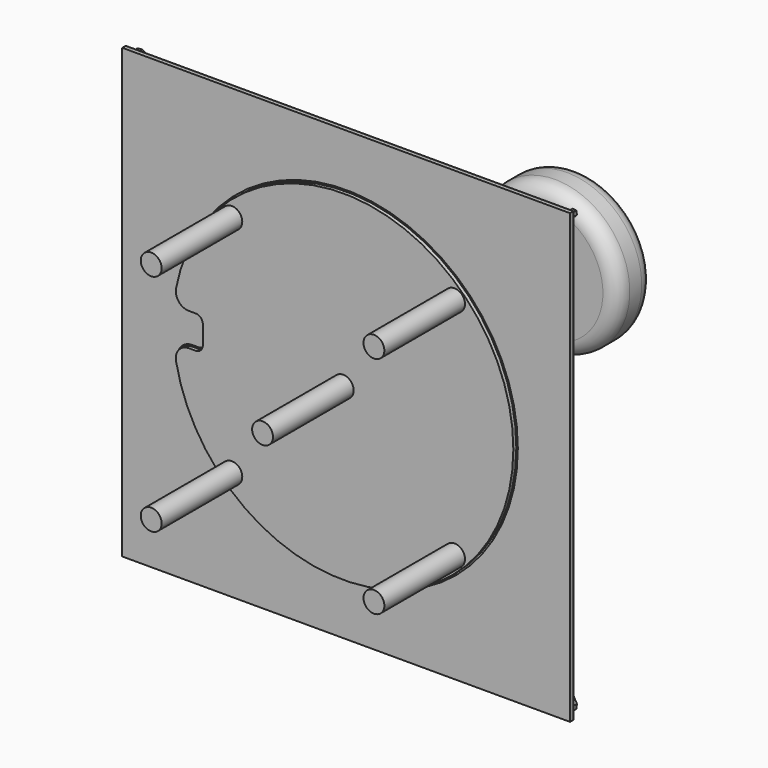
from build123d import *

# Parameters (mm, degrees)
F0_W      = 150
F0_H      = 150
F1_DEPTH  = 2.5
F2_R      = 15
F3_DEPTH  = 30
F4_T      = 4.5
F5_R      = 3.5
F6_DEPTH  = 35
F7_R      = 1.5
F10_DEPTH = 25
F11_R     = 3.5
F12_DEPTH = 35
F16_COUNT = 4
F18_DEPTH = 1.25
F20_DEPTH = 1.25
F21_R     = 10
F22_DEPTH = 80
F23_R     = 25
F24_DEPTH = 15
F25_R     = 5


# Not quite as in the source:
# - a fillet or chamfer that OpenCascade refuses, or shapes differently, is made with other operations: its cross-section is extruded or revolved along the edge and cut away or added
# - a shell that OpenCascade refuses in one call is made with other operations: the cavity is built on its own and cut out


with BuildPart() as f1:
    # F0 (on Front) → F1 (new body)
    with BuildSketch(Plane.XZ):
        Rectangle(F0_W, F0_H)
    extrude(amount=F1_DEPTH)

    # F2 (on face) → F3 (join)
    with BuildSketch(Plane(origin=(0, 0, 0), x_dir=(-1, 0, 0), z_dir=(0, 1, 0))):
        Circle(F2_R)
    extrude(amount=F3_DEPTH)

    # F4: shell of thickness 4.5, made by hand


with BuildPart() as f4_core1:
    # F4_t2: copy of F1
    add(f1.part)

    # the walls: a layer under each face that stays
    f4_faces = [f4_core1.faces().sort_by_distance(p)[0] for p in [
        (75, -1.25, 0),
        (0, -1.25, -75),
        (0, -1.25, 75),
        (0, -2.5, 0),
        (-75, -1.25, 0),
        (15, 15, 0),
    ]]
    thicken(f4_faces, amount=-F4_T, mode=Mode.SUBTRACT)


with BuildPart() as f1_1:
    add(f1.part)

    # what is left inside the walls is the cavity
    f4_cavity = [f4_core1.part.solids().sort_by_distance(p)[0] for p in [
        (10.455, 20.666667, 0),
    ]]
    add(f4_cavity, mode=Mode.SUBTRACT)

    # F7
    f7_edges = [f1_1.edges().sort_by_distance(p)[0] for p in [
        (75, 0, 0),
        (0, 0, -75),
        (0, 0, 75),
        (-75, 0, 0),
        (15, 0, 0),
    ]]
    fillet(f7_edges, radius=F7_R)

    # F8: fillet of radius 5 on 1 edges, made by hand

    # F8_s1 → F8_t2 (revolve, cut)
    with BuildSketch(Plane.XY):
        with BuildLine():
            ThreePointArc((-15, 25.0250628145), (-13.7080992435, 28.3791647807), (-10.5, 30))
            Line((-10.5, 30), (-15, 30))
            Line((-15, 30), (-15, 25.0250628145))
        make_face()
    revolve(axis=Axis((0, 30, 0), (0, 1, 0)), mode=Mode.SUBTRACT)

    # F17 (on face) → F18 (cut)
    with BuildSketch(Plane.XZ.offset(2.5)):
        with BuildLine():
            ThreePointArc((-51.5388203202, -5), (-55.3964040693, -6.8189549486), (-56.4472793983, -10.9523809524))
            ThreePointArc((-56.4472793983, -10.9523809524), (57.5, 0), (-56.4472793983, 10.9523809524))
            ThreePointArc((-56.4472793983, 10.9523809524), (-55.3964040693, 6.8189549486), (-51.5388203202, 5))
            Line((-51.5388203202, 5), (-49.5, 5))
            ThreePointArc((-49.5, 5), (-48.0857864376, 4.4142135624), (-47.5, 3))
            Line((-47.5, 3), (-47.5, -3))
            ThreePointArc((-47.5, -3), (-48.0857864376, -4.4142135624), (-49.5, -5))
            Line((-49.5, -5), (-51.5388203202, -5))
        make_face()
    extrude(amount=-F18_DEPTH, mode=Mode.SUBTRACT)

    # F21 (on face) → F22 (join)
    with BuildSketch(Plane.XZ):
        Circle(F21_R)
    extrude(amount=-F22_DEPTH)

    # F23 (on face) → F24 (join)
    with BuildSketch(Plane(origin=(0, 80, 0), x_dir=(-1, 0, 0), z_dir=(0, 1, 0))):
        Circle(F23_R)
    extrude(amount=F24_DEPTH)

    # F25
    f25_edges = [f1_1.edges().sort_by_distance(p)[0] for p in [
        (25, 95, 0),
        (25, 80, 0),
    ]]
    fillet(f25_edges, radius=F25_R)


with BuildPart() as f6:
    # F5 (on face) → F6 (new body)
    with BuildSketch(Plane.XZ.offset(2.5)):
        with Locations((-37.2992306948, -37.6147218049)):
            Circle(F5_R)
    extrude(amount=F6_DEPTH)


with BuildPart() as f6b:
    # F5 (on face) → F6, piece 2 (new body)
    with BuildSketch(Plane.XZ.offset(2.5)):
        with Locations((37.2992306948, -37.6147218049)):
            Circle(F5_R)
    extrude(amount=F6_DEPTH)


with BuildPart() as f6c:
    # F5 (on face) → F6, piece 3 (new body)
    with BuildSketch(Plane.XZ.offset(2.5)):
        with Locations((-37.2992306948, 37.6147218049)):
            Circle(F5_R)
    extrude(amount=F6_DEPTH)


with BuildPart() as f6d:
    # F5 (on face) → F6, piece 4 (new body)
    with BuildSketch(Plane.XZ.offset(2.5)):
        with Locations((37.2992306948, 37.6147218049)):
            Circle(F5_R)
    extrude(amount=F6_DEPTH)


with BuildPart() as f10:
    # F9 (on face) → F10 (new body)
    with BuildSketch(Plane(origin=(0, 0, 0), x_dir=(-1, 0, 0), z_dir=(0, 1, 0))):
        with BuildLine():
            Line((73.5, -73.5), (73.5, -72.0857864376))
            Line((73.5, -72.0857864376), (12.35292148, -10.9387079177))
            ThreePointArc((12.35292148, -10.9387079177), (11.6672618896, -11.6672618896), (10.9387079177, -12.35292148))
            Line((10.9387079177, -12.35292148), (72.0857864376, -73.5))
            Line((72.0857864376, -73.5), (73.5, -73.5))
        make_face()
        with BuildLine():
            ThreePointArc((10.9387079177, -12.35292148), (11.6672618896, -11.6672618896), (12.35292148, -10.9387079177))
            Line((12.35292148, -10.9387079177), (11.2901120254, -9.8758984631))
            ThreePointArc((11.2901120254, -9.8758984631), (10.6066017178, -10.6066017178), (9.8758984631, -11.2901120254))
            Line((9.8758984631, -11.2901120254), (10.9387079177, -12.35292148))
        make_face()
    extrude(amount=F10_DEPTH)

    # F14 (on mid) → F15 (revolve, cut)
    with BuildSketch(Plane(origin=(0, 0, 0), x_dir=(0, -1, 0), z_dir=(-0.7071067812, 0, 0.7071067812))):
        Polygon((-25, -15), (-25, -103.9446968344), (-2, -103.9446968344), align=None)
    revolve(axis=Axis((0, 0, 0), (0, -1, 0)), mode=Mode.SUBTRACT)


with BuildPart() as f12:
    # F11 (on face) → F12 (new body)
    with BuildSketch(Plane.XZ.offset(2.5)):
        Circle(F11_R)
    extrude(amount=F12_DEPTH)


with BuildPart() as f16_1:
    # F16: instance of F10
    add(f10.part.rotate(Axis((0, 0, 0), (0, -1, 0)), 1 * 360 / F16_COUNT))


with BuildPart() as f16_2:
    # F16: instance of F10
    add(f10.part.rotate(Axis((0, 0, 0), (0, -1, 0)), 2 * 360 / F16_COUNT))


with BuildPart() as f16_3:
    # F16: instance of F10
    add(f10.part.rotate(Axis((0, 0, 0), (0, -1, 0)), 3 * 360 / F16_COUNT))


with BuildPart() as f20:
    # F19 (on face) → F20 (new body)
    with BuildSketch(Plane.XZ.offset(2.5)):
        with BuildLine():
            ThreePointArc((-51.6599457994, -5.5), (-55.0513910873, -7.0967699239), (-55.9813100868, -10.7281368821))
            ThreePointArc((-55.9813100868, -10.7281368821), (57, 0), (-55.9813100868, 10.7281368821))
            ThreePointArc((-55.9813100868, 10.7281368821), (-55.0513910873, 7.0967699239), (-51.6599457994, 5.5))
            Line((-51.6599457994, 5.5), (-49.4, 5.5))
            ThreePointArc((-49.4, 5.5), (-47.7029437252, 4.7970562748), (-47, 3.1))
            Line((-47, 3.1), (-47, -3.1))
            ThreePointArc((-47, -3.1), (-47.7029437252, -4.7970562748), (-49.4, -5.5))
            Line((-49.4, -5.5), (-51.6599457994, -5.5))
        make_face()
    extrude(amount=F20_DEPTH)


solid = Compound([f1_1.part, f6.part, f6b.part, f6c.part, f6d.part, f10.part, f12.part, f16_1.part, f16_2.part, f16_3.part, f20.part])
